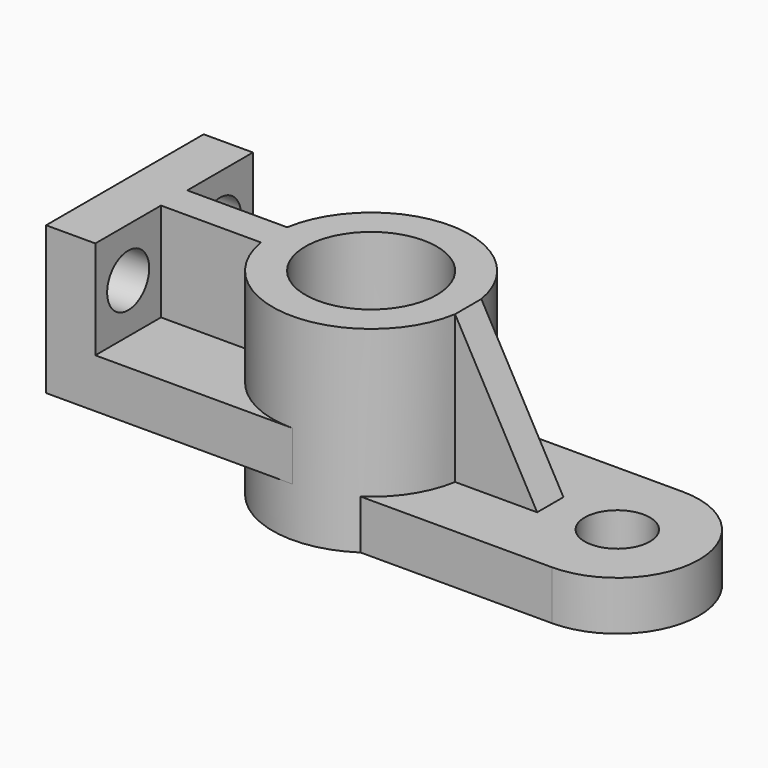
from build123d import *

# Parameters (mm, degrees)
F0_R      = 30
F0_R_2    = 20
F1_DEPTH  = 60
F2_R      = 20
F2_R_2    = 9.9351128524
F3_DEPTH  = 15
F5_DEPTH  = 45
F6_SIZE2  = 24.99999
F6_SIZE   = 44.99999
F7_R      = 20
F8_DEPTH  = 15
F10_DEPTH = 30
F11_R     = 8
F12_DEPTH = 15


# Not quite as in the source:
# - a fillet or chamfer is up to 0.001 mm smaller than in the source, because OpenCascade refuses the exact size


with BuildPart() as f1:
    # F0 (on Top) → F1 (new body)
    with BuildSketch(Plane.XY):
        Circle(F0_R)
        Circle(F0_R_2, mode=Mode.SUBTRACT)
    extrude(amount=F1_DEPTH)

    # F2 (on Top) → F3 (join)
    with BuildSketch(Plane.XY):
        with BuildLine():
            Line((16.7213538347, -24.9077563409), (75, -24.9077563409))
            ThreePointArc((75, -24.9077563409), (99.9077563409, 0), (75, 24.9077563409))
            Line((75, 24.9077563409), (16.7213538347, 24.9077563409))
            ThreePointArc((16.7213538347, 24.9077563409), (-30, 0), (16.7213538347, -24.9077563409))
        make_face()
        Circle(F2_R, mode=Mode.SUBTRACT)
        with Locations((75, 0)):
            Circle(F2_R_2, mode=Mode.SUBTRACT)
    extrude(amount=F3_DEPTH)

    # F4 (on face) → F5 (join, through all)
    with BuildSketch(Plane.XY.offset(15)):
        with BuildLine():
            Line((54.5803989155, 5), (29.5803989155, 5))
            ThreePointArc((29.5803989155, 5), (30, 0), (29.5803989155, -5))
            Line((29.5803989155, -5), (54.5803989155, -5))
            Line((54.5803989155, -5), (54.5803989155, 5))
        make_face()
    extrude(amount=F5_DEPTH)

    # F6 (size 45 and 25 in the source; OpenCascade refuses exactly that, so slightly less here)
    f6_edges = [f1.edges().sort_by_distance(p)[0] for p in [
        (54.580399, 0, 60),
    ]]
    f6_side = f1.faces().sort_by_distance((54.580399, 0, 37.5))[0]
    chamfer(f6_edges, length=F6_SIZE, length2=F6_SIZE2, reference=f6_side)

    # F7 (on face) → F8 (join)
    with BuildSketch(Plane.XY.offset(15)):
        with BuildLine():
            Line((29.5803989155, -5), (29.5803989155, 5))
            ThreePointArc((29.5803989155, 5), (19.364916731, 22.9128784748), (0, 30))
            ThreePointArc((0, 30), (-30, 0), (0, -30))
            ThreePointArc((0, -30), (19.364916731, -22.9128784748), (29.5803989155, -5))
        make_face()
        Circle(F7_R, mode=Mode.SUBTRACT)
        with BuildLine():
            ThreePointArc((0, -30), (-30, 0), (0, 30))
            Line((0, 30), (-75, 30))
            Line((-75, 30), (-75, -30))
            Line((-75, -30), (0, -30))
        make_face()
    extrude(amount=F8_DEPTH)

    # F9 (on face) → F10 (join, through all)
    with BuildSketch(Plane.XY.offset(30)):
        with BuildLine():
            Line((-60, 30), (-75, 30))
            Line((-75, 30), (-75, -30))
            Line((-75, -30), (-60, -30))
            Line((-60, -30), (-60, -5))
            Line((-60, -5), (-29.5803989155, -5))
            ThreePointArc((-29.5803989155, -5), (-30, 0), (-29.5803989155, 5))
            Line((-29.5803989155, 5), (-60, 5))
            Line((-60, 5), (-60, 30))
        make_face()
    extrude(amount=F10_DEPTH)

    # F11 (on face) → F12 (cut, through all)
    with BuildSketch(Plane(origin=(-75, 0, 0), x_dir=(0, -1, 0), z_dir=(-1, 0, 0))):
        with Locations((17.5, 45)):
            Circle(F11_R)
        with Locations((-17.5, 45)):
            Circle(F11_R)
    extrude(amount=-F12_DEPTH, mode=Mode.SUBTRACT)


solid = f1.part
